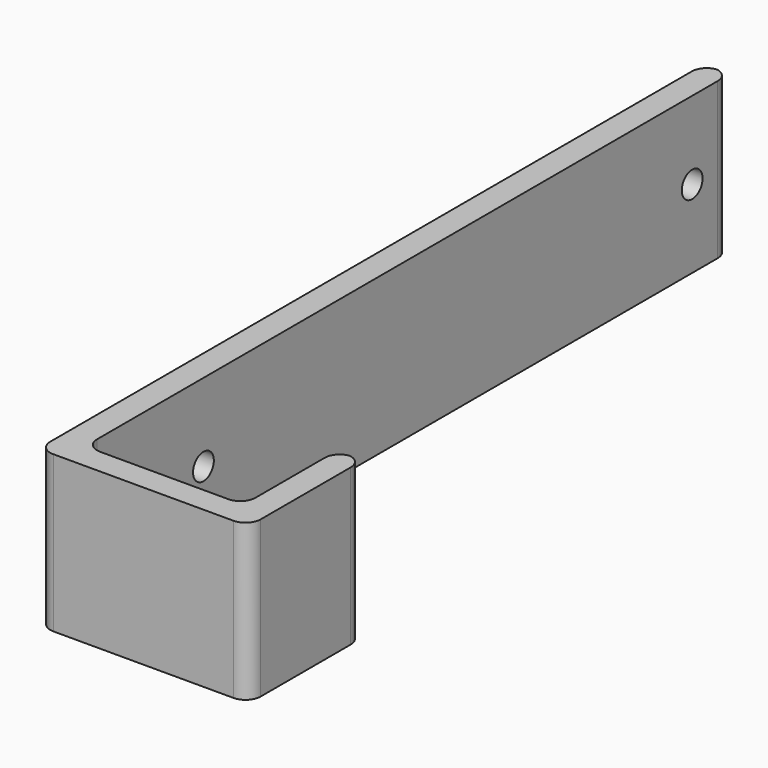
from build123d import *

# Parameters (mm, degrees)
F0_W        = 38.6806862377
F0_H        = 6.35
F1_DEPTH    = 38.1
F2_T1_DEPTH = 38.1
F2_T3_DEPTH = 56.4963073453
F3_R        = 3.175
F4_DEPTH    = 25.4


# Not quite as in the source:
# - a fillet or chamfer that OpenCascade refuses, or shapes differently, is made with other operations: its cross-section is extruded or revolved along the edge and cut away or added


with BuildPart() as f1:
    # F0 (on Top) → F1 (new body)
    with BuildSketch(Plane.XY):
        Polygon((-10.8904888918, 145.4896045446), (-17.2404888918, 145.4896045446), (-17.2404888918, -57.7103954554), (-10.8904888918, -57.7103954554), (-10.8904888918, -51.3603954554), align=None)
        with Locations((8.449854227, -54.5353954554)):
            Rectangle(F0_W, F0_H)
        Polygon((27.7901973458, -22.8552754367), (27.7901973458, -51.3603954554), (27.7901973458, -57.7103954554), (34.1401973458, -57.7103954554), (34.1401973458, -22.8552754367), align=None)
    extrude(amount=F1_DEPTH)

    # F2: fillet of radius 3.6792614691 on 8 edges, made by hand

    # F2_s2 → F2_t1 (join)
    with BuildSketch(Plane.XY):
        with BuildLine():
            ThreePointArc((-7.2112274228, -51.3603954554), (-9.8128581573, -50.2827647208), (-10.8904888918, -47.6811339863))
            Line((-10.8904888918, -47.6811339863), (-10.8904888918, -51.3603954554))
            Line((-10.8904888918, -51.3603954554), (-7.2112274228, -51.3603954554))
        make_face()
        with BuildLine():
            ThreePointArc((27.7901973458, -47.6811339863), (26.7125666113, -50.2827647208), (24.1109358768, -51.3603954554))
            Line((24.1109358768, -51.3603954554), (27.7901973458, -51.3603954554))
            Line((27.7901973458, -51.3603954554), (27.7901973458, -47.6811339863))
        make_face()
    extrude(amount=F2_T1_DEPTH)

    # F2_s4 → F2_t3 (cut)
    with BuildSketch(Plane.XY.offset(-9.1981536726)):
        with BuildLine():
            ThreePointArc((31.4694588149, -22.8552754367), (28.8678280803, -23.9329061712), (27.7901973458, -26.5345369057))
            Line((27.7901973458, -26.5345369057), (27.7901973458, -22.8552754367))
            Line((27.7901973458, -22.8552754367), (31.4694588149, -22.8552754367))
        make_face()
        with BuildLine():
            ThreePointArc((34.1401973458, -26.5345369057), (33.0625666113, -23.9329061712), (30.4609358768, -22.8552754367))
            Line((30.4609358768, -22.8552754367), (34.1401973458, -22.8552754367))
            Line((34.1401973458, -22.8552754367), (34.1401973458, -26.5345369057))
        make_face()
        with BuildLine():
            ThreePointArc((-17.2404888918, -54.0311339863), (-16.1628581573, -56.6327647208), (-13.5612274228, -57.7103954554))
            Line((-13.5612274228, -57.7103954554), (-17.2404888918, -57.7103954554))
            Line((-17.2404888918, -57.7103954554), (-17.2404888918, -54.0311339863))
        make_face()
        with BuildLine():
            ThreePointArc((30.4609358768, -57.7103954554), (33.0625666113, -56.6327647208), (34.1401973458, -54.0311339863))
            Line((34.1401973458, -54.0311339863), (34.1401973458, -57.7103954554))
            Line((34.1401973458, -57.7103954554), (30.4609358768, -57.7103954554))
        make_face()
        with BuildLine():
            ThreePointArc((-14.5697503609, 145.4896045446), (-11.9681196264, 144.4119738101), (-10.8904888918, 141.8103430756))
            Line((-10.8904888918, 141.8103430756), (-10.8904888918, 145.4896045446))
            Line((-10.8904888918, 145.4896045446), (-14.5697503609, 145.4896045446))
        make_face()
        with BuildLine():
            ThreePointArc((-13.5612274228, 145.4896045446), (-16.1628581573, 144.4119738101), (-17.2404888918, 141.8103430756))
            Line((-17.2404888918, 141.8103430756), (-17.2404888918, 145.4896045446))
            Line((-17.2404888918, 145.4896045446), (-13.5612274228, 145.4896045446))
        make_face()
    extrude(amount=F2_T3_DEPTH, mode=Mode.SUBTRACT)

    # F3 (on face) → F4 (cut)
    with BuildSketch(Plane(origin=(-17.2404888918, 0, 0), x_dir=(0, -1, 0), z_dir=(-1, 0, 0))):
        with Locations((-134.0196450753, 19.05)):
            Circle(F3_R)
        with Locations((15.2053549247, 19.05)):
            Circle(F3_R)
    extrude(amount=-F4_DEPTH, mode=Mode.SUBTRACT)


solid = f1.part
